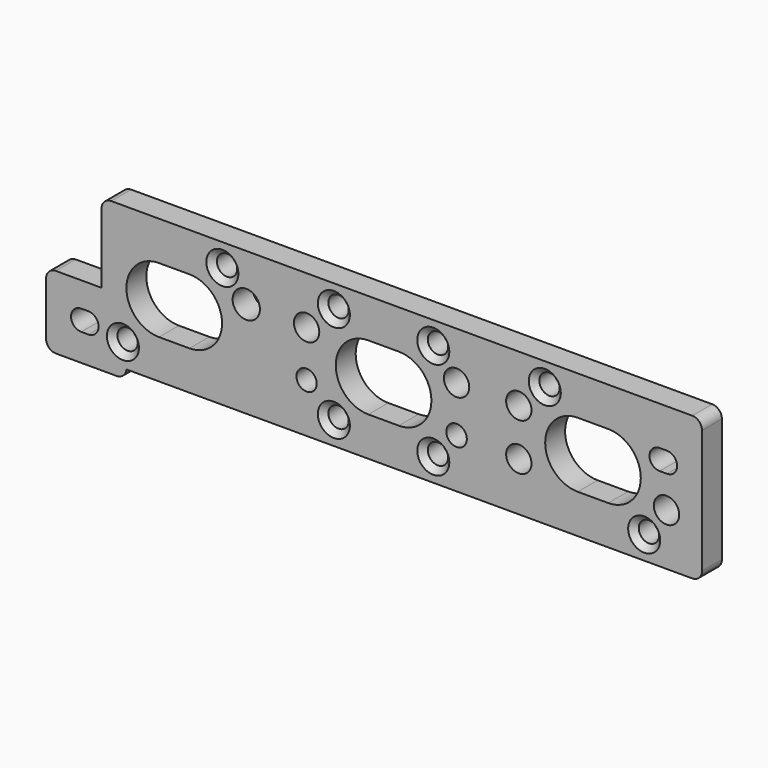
from build123d import *

# Parameters (mm, degrees)
F2_DEPTH    = 12.75
F0_R        = 7
F0_R_2      = 6.5
F0_R_3      = 5.2
F0_R_4      = 5.25
F3_DEPTH    = 25
F4_T1_DEPTH = 37.75
F4_T3_DEPTH = 37.6621075041
F5_R        = 5.207
F6_DEPTH    = 25
F7_SIZE     = 3


# Not quite as in the source:
# - a fillet or chamfer that OpenCascade refuses, or shapes differently, is made with other operations: its cross-section is extruded or revolved along the edge and cut away or added


with BuildPart() as f2:
    # F1 (on Front) → F2 (new body)
    with BuildSketch(Plane.XZ):
        Polygon((270.335, 36.6037324816), (-37.1999023023, 36.6037324816), (-37.1999023023, -4.1193680316), (-65.5964598894, -4.1193680316), (-65.5964598894, -41.3573689769), (-24.4499023023, -41.3573689769), (-24.4499023023, -36.7762675184), (270.335, -36.7762675184), align=None)
    extrude(amount=F2_DEPTH)

    # F0 (on Front) → F3 (cut)
    with BuildSketch(Plane.XZ):
        with BuildLine():
            Line((7.8300976977, 16.6037324816), (-7.7599023023, 16.6037324816))
            ThreePointArc((-7.7599023023, 16.6037324816), (-24.4499023023, -0.0862675184), (-7.7599023023, -16.7762675184))
            Line((-7.7599023023, -16.7762675184), (7.8300976977, -16.7762675184))
            ThreePointArc((7.8300976977, -16.7762675184), (24.5200976977, -0.0862675184), (7.8300976977, 16.6037324816))
        make_face()
        with BuildLine():
            Line((115.045, 16.6037324816), (99.455, 16.6037324816))
            ThreePointArc((99.455, 16.6037324816), (82.765, -0.0862675184), (99.455, -16.7762675184))
            Line((99.455, -16.7762675184), (115.045, -16.7762675184))
            ThreePointArc((115.045, -16.7762675184), (131.735, -0.0862675184), (115.045, 16.6037324816))
        make_face()
        with BuildLine():
            Line((222.295, 16.6037324816), (206.705, 16.6037324816))
            ThreePointArc((206.705, 16.6037324816), (190.015, -0.0862675184), (206.705, -16.7762675184))
            Line((206.705, -16.7762675184), (222.295, -16.7762675184))
            ThreePointArc((222.295, -16.7762675184), (238.985, -0.0862675184), (222.295, 16.6037324816))
        make_face()
        with Locations((36.93, 12.5237324816)):
            Circle(F0_R)
        with Locations((67.822315464, 12.1637324816)):
            Circle(F0_R_2)
        with Locations((67.822315464, -11.5762675184)):
            Circle(F0_R_3)
        with BuildLine():
            Line((-43.9464598894, -16.8693680316), (-47.5964598894, -16.8693680316))
            ThreePointArc((-47.5964598894, -16.8693680316), (-52.8464598894, -22.1193680316), (-47.5964598894, -27.3693680316))
            Line((-47.5964598894, -27.3693680316), (-43.9464598894, -27.3693680316))
            ThreePointArc((-43.9464598894, -27.3693680316), (-38.6964598894, -22.1193680316), (-43.9464598894, -16.8693680316))
        make_face()
        with Locations((144.635, 12.2237324816)):
            Circle(F0_R_2)
        with Locations((144.635, -11.5262675184)):
            Circle(F0_R_4)
        with Locations((176.515, 12.2237324816)):
            Circle(F0_R_2)
        with Locations((176.515, -11.7762675184)):
            Circle(F0_R_2)
        with BuildLine():
            Line((252.38, 16.6037324816), (248.64, 16.6037324816))
            ThreePointArc((248.64, 16.6037324816), (243.435, 11.3987324816), (248.64, 6.1937324816))
            Line((248.64, 6.1937324816), (252.38, 6.1937324816))
            ThreePointArc((252.38, 6.1937324816), (257.585, 11.3987324816), (252.38, 16.6037324816))
        make_face()
        with Locations((252.155, -10.2762675184)):
            Circle(F0_R_2)
    extrude(amount=F3_DEPTH, mode=Mode.SUBTRACT)

    # F4: fillet of radius 5 on 6 edges, made by hand

    # F4_s2 → F4_t1 (cut)
    with BuildSketch(Plane.XZ.offset(-12.5)):
        with BuildLine():
            ThreePointArc((-32.1999023023, 36.6037324816), (-35.7354362082, 35.1392663875), (-37.1999023023, 31.6037324816))
            Line((-37.1999023023, 31.6037324816), (-37.1999023023, 36.6037324816))
            Line((-37.1999023023, 36.6037324816), (-32.1999023023, 36.6037324816))
        make_face()
        with BuildLine():
            ThreePointArc((-60.5964598894, -4.1193680316), (-64.1319937953, -5.5838341257), (-65.5964598894, -9.1193680316))
            Line((-65.5964598894, -9.1193680316), (-65.5964598894, -4.1193680316))
            Line((-65.5964598894, -4.1193680316), (-60.5964598894, -4.1193680316))
        make_face()
        with BuildLine():
            ThreePointArc((-60.5964598894, -41.3573689769), (-64.1319937953, -39.8929028828), (-65.5964598894, -36.3573689769))
            Line((-65.5964598894, -36.3573689769), (-65.5964598894, -41.3573689769))
            Line((-65.5964598894, -41.3573689769), (-60.5964598894, -41.3573689769))
        make_face()
        with BuildLine():
            ThreePointArc((270.335, 31.6037324816), (268.8705339059, 35.1392663875), (265.335, 36.6037324816))
            Line((265.335, 36.6037324816), (270.335, 36.6037324816))
            Line((270.335, 36.6037324816), (270.335, 31.6037324816))
        make_face()
        with BuildLine():
            ThreePointArc((270.335, -31.7762675184), (268.8705339059, -35.3118014243), (265.335, -36.7762675184))
            Line((265.335, -36.7762675184), (270.335, -36.7762675184))
            Line((270.335, -36.7762675184), (270.335, -31.7762675184))
        make_face()
    extrude(amount=F4_T1_DEPTH, mode=Mode.SUBTRACT)

    # F4_s4 → F4_t3 (cut)
    with BuildSketch(Plane.XZ.offset(-12.4560537521)):
        with BuildLine():
            ThreePointArc((-24.4499023023, -36.7762675184), (-26.0481320759, -40.03802739), (-29.4323238031, -41.3573689769))
            Line((-29.4323238031, -41.3573689769), (-24.4499023023, -41.3573689769))
            Line((-24.4499023023, -41.3573689769), (-24.4499023023, -36.7762675184))
        make_face()
    extrude(amount=F4_T3_DEPTH, mode=Mode.SUBTRACT)

    # F5 (on Front) → F6 (cut)
    with BuildSketch(Plane.XZ):
        with Locations((132.714, 24.968)):
            Circle(F5_R)
        with Locations((132.714, -24.968)):
            Circle(F5_R)
        with Locations((81.786, -24.968)):
            Circle(F5_R)
        with Locations((81.786, 24.968)):
            Circle(F5_R)
        with Locations((240.74, -24.968)):
            Circle(F5_R)
        with Locations((-26.24, -24.968)):
            Circle(F5_R)
        with Locations((24.687, 24.968)):
            Circle(F5_R)
        with Locations((189.813, 24.968)):
            Circle(F5_R)
    extrude(amount=F6_DEPTH, mode=Mode.SUBTRACT)

    # F7
    f7_edges = [f2.edges().sort_by_distance(p)[0] for p in [
        (19.48, -12.75, 24.968),
        (-31.447, -12.75, -24.968),
        (76.579, -12.75, 24.968),
        (127.507, -12.75, 24.968),
        (127.507, -12.75, -24.968),
        (76.579, -12.75, -24.968),
        (184.606, -12.75, 24.968),
        (235.533, -12.75, -24.968),
    ]]
    chamfer(f7_edges, length=F7_SIZE)


solid = f2.part
